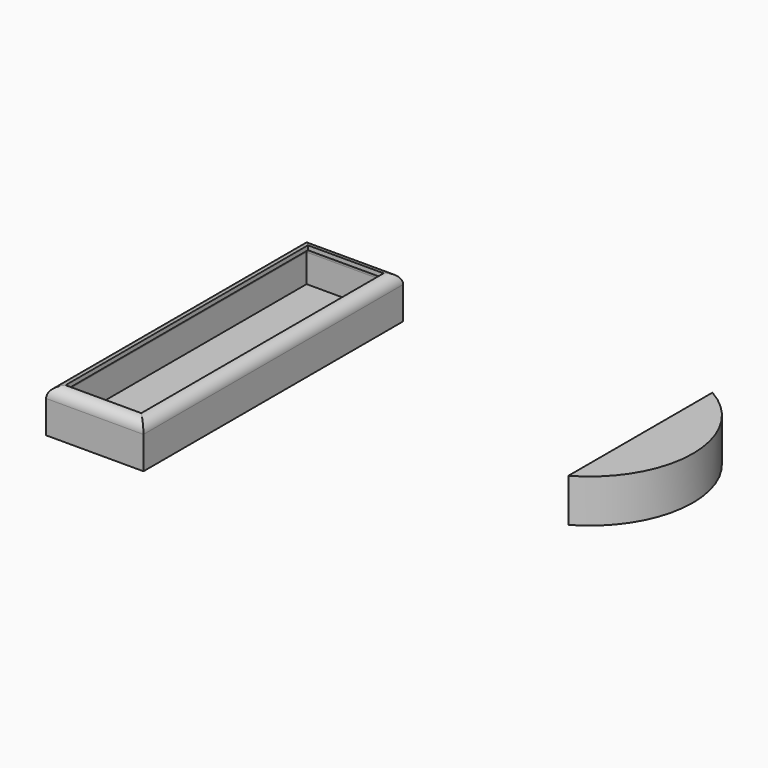
from build123d import *

# Parameters (mm, degrees)
F0_W     = 90
F0_H     = 300
F1_DEPTH = 40
F2_R     = 10
F3_T     = -4
F5_DEPTH = 40


# Not quite as in the source:
# - a shell that OpenCascade refuses in one call is made with other operations: the cavity is built on its own and cut out


with BuildPart() as f1:
    # F0 (on Top) → F1 (new body)
    with BuildSketch(Plane.XY):
        with Locations((-135.0600157978, -97.4264368415)):
            Rectangle(F0_W, F0_H)
    extrude(amount=F1_DEPTH)

    # F2
    f2_edges = [f1.edges().sort_by_distance(p)[0] for p in [
        (-90.060016, -97.426437, 40),
        (-135.060016, -247.426437, 40),
        (-180.060016, -97.426437, 40),
        (-135.060016, 52.573563, 40),
    ]]
    fillet(f2_edges, radius=F2_R)

    # F3: a shell. OpenCascade refuses it in one call, so the cavity is built on its own and cut out:
    # the body offset inwards by the wall thickness, plus a prism from it out through each open face.
    f3_core = offset(f1.part, amount=F3_T, mode=Mode.PRIVATE)
    f3_exits = [f3_core.faces().sort_by_distance(p)[0] for p in [
        (-135.060016, -97.426437, 36),
    ]]
    add(f3_core, mode=Mode.SUBTRACT)
    extrude(f3_exits, amount=-F3_T, mode=Mode.SUBTRACT)


with BuildPart() as f5:
    # F4 (on Top) → F5 (new body)
    with BuildSketch(Plane.XY):
        with BuildLine():
            Line((201.7689708893, 45.1520286221), (201.7689708893, -121.3005959367))
            ThreePointArc((201.7689708893, -121.3005959367), (250.3483896515, -38.0742836573), (201.7689708893, 45.1520286221))
        make_face()
    extrude(amount=F5_DEPTH)


solid = Compound([f1.part, f5.part])
